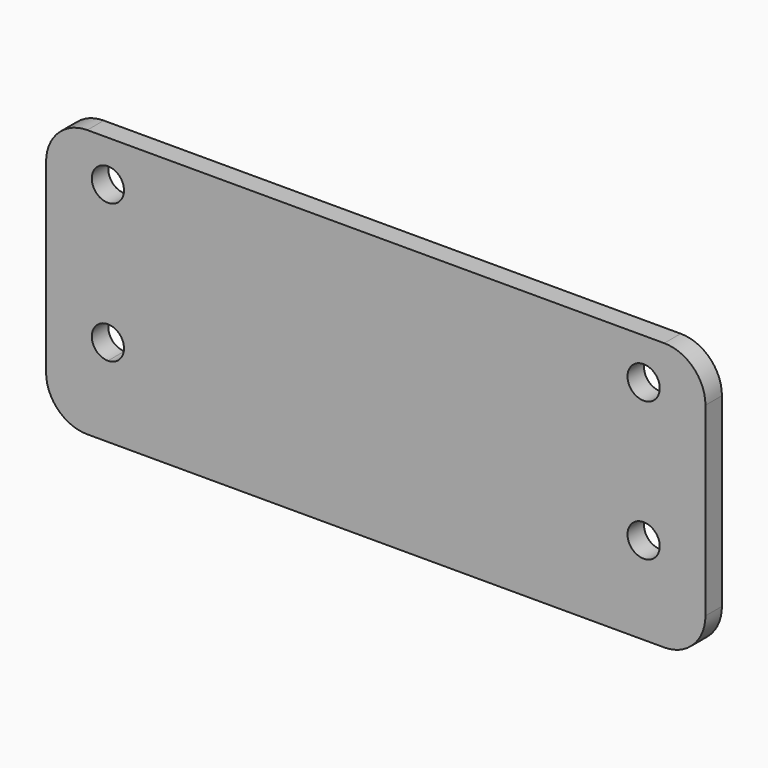
from build123d import *

# Parameters (mm, degrees)
F0_R     = 4.9657
F0_W     = 101.6
F0_H     = 82.55
F1_DEPTH = 3.175
F2_R     = 12.7


with BuildPart() as f1:
    # F0 (on Front) → F1 (new body, symmetric)
    with BuildSketch(Plane.XZ):
        Polygon((-82.55, 0), (0, 0), (0, 82.55), (-101.6, 82.55), (-101.6, 0), align=None)
        with BuildLine():
            ThreePointArc((-77.5843, 26.9875), (-79.0387198567, 23.4762198567), (-82.55, 22.0218))
            ThreePointArc((-82.55, 22.0218), (-87.5157, 26.9875), (-82.55, 31.9532))
            ThreePointArc((-82.55, 31.9532), (-79.0387198567, 30.4987801433), (-77.5843, 26.9875))
        make_face(mode=Mode.SUBTRACT)
        with Locations((-82.55, 69.85)):
            Circle(F0_R, mode=Mode.SUBTRACT)
        with Locations((50.8, 41.275)):
            Rectangle(F0_W, F0_H)
        with Locations((82.55, 26.9875)):
            Circle(F0_R, mode=Mode.SUBTRACT)
        with Locations((82.55, 69.85)):
            Circle(F0_R, mode=Mode.SUBTRACT)
    extrude(amount=F1_DEPTH, both=True)

    # F2
    f2_edges = [f1.edges().sort_by_distance(p)[0] for p in [
        (-101.6, 0, 82.55),
        (101.6, 0, 0),
        (101.6, 0, 82.55),
        (-101.6, 0, 0),
    ]]
    fillet(f2_edges, radius=F2_R)


solid = f1.part
